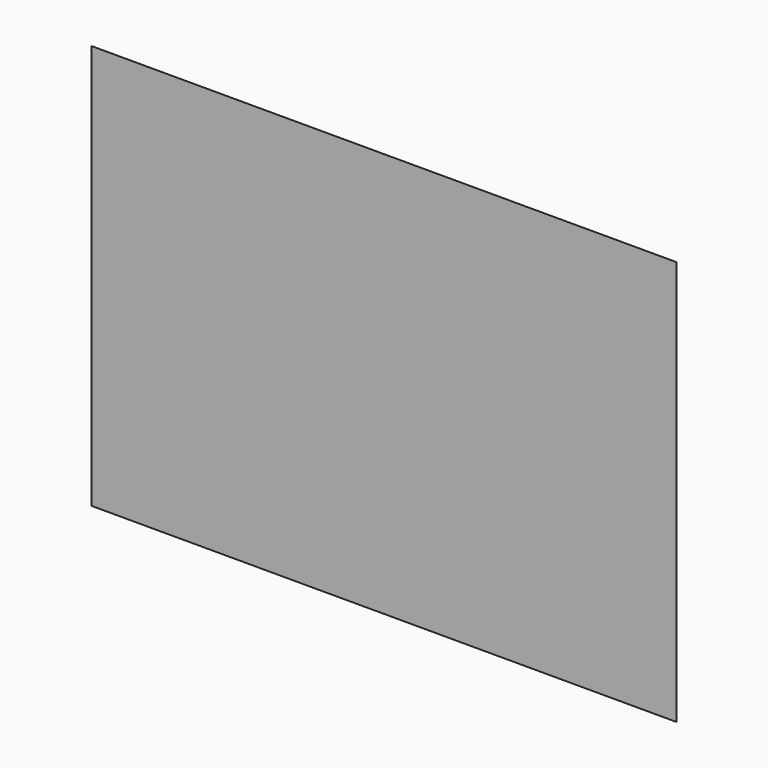
from build123d import *

# Parameters (mm, degrees)
F1_W     = 330.2
F1_H     = 228.6
F2_DEPTH = 10
F3_SIZE  = 9.99999


# Not quite as in the source:
# - a fillet or chamfer is up to 0.001 mm smaller than in the source, because OpenCascade refuses the exact size


with BuildPart() as f2:
    # F1 (on face) → F2 (new body)
    with BuildSketch(Plane.XZ):
        Rectangle(F1_W, F1_H)
    extrude(amount=F2_DEPTH)

    # F3 (size 10 in the source; OpenCascade refuses exactly that, so slightly less here)
    f3_edges = [f2.edges().sort_by_distance(p)[0] for p in [
        (0, 0, 114.3),
        (165.1, 0, 0),
        (-165.1, 0, 0),
        (0, 0, -114.3),
    ]]
    chamfer(f3_edges, length=F3_SIZE)


solid = f2.part
